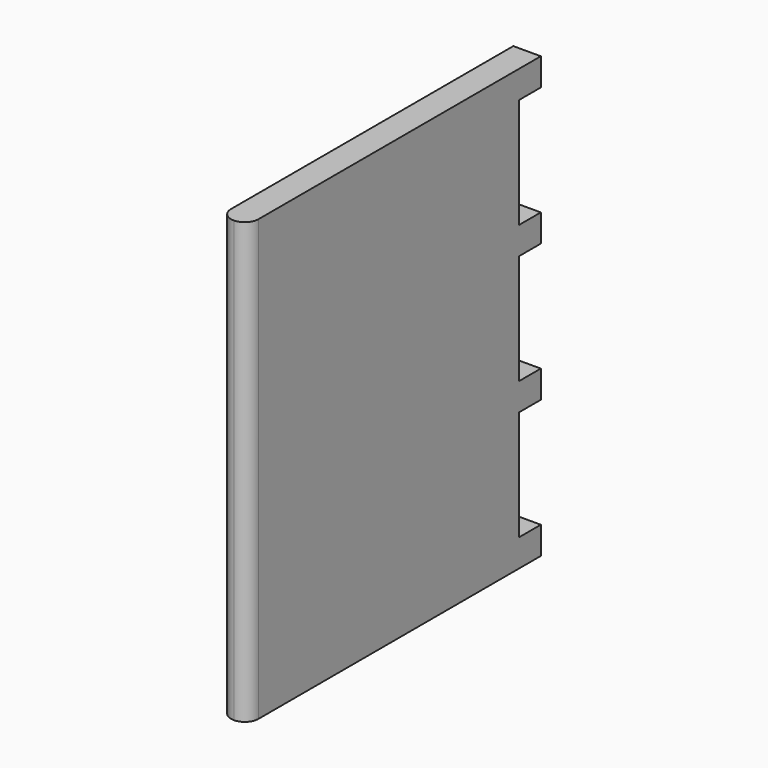
from build123d import *

# Parameters (mm, degrees)
F0_W     = 254
F0_H     = 304.8
F1_DEPTH = 9.525
F2_R     = 9.52499
F3_W     = 19.05
F3_H     = 76.2
F4_DEPTH = 19.051


# Not quite as in the source:
# - a fillet or chamfer is up to 0.001 mm smaller than in the source, because OpenCascade refuses the exact size
# - a feature names something its author has since deleted; it is built from what else it names


with BuildPart() as f1:
    # F0 (on Right) → F1 (new body, symmetric)
    with BuildSketch(Plane.YZ):
        Rectangle(F0_W, F0_H)
    extrude(amount=F1_DEPTH, both=True)

    # F2 (radius 9.525 in the source; OpenCascade refuses exactly that, so slightly less here)
    f2_edges = [f1.edges().sort_by_distance(p)[0] for p in [
        (9.525, -127, 0),
        (-9.525, -127, 0),
    ]]
    fillet(f2_edges, radius=F2_R)

    # F3 (on face) → F4 (cut, through all)
    with BuildSketch(Plane.YZ.offset(9.525)):
        with Locations((117.475, 95.25)):
            Rectangle(F3_W, F3_H)
        with Locations((117.475, 0)):
            Rectangle(F3_W, F3_H)
        with Locations((117.475, -95.25)):
            Rectangle(F3_W, F3_H)
    extrude(amount=-F4_DEPTH, mode=Mode.SUBTRACT)


solid = f1.part
